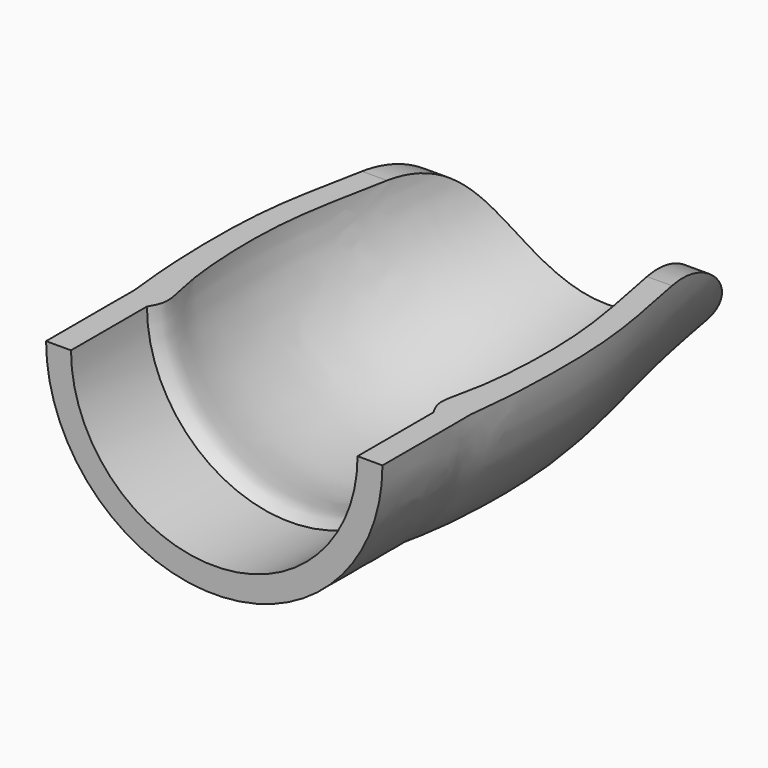
from build123d import *

# Parameters (mm, degrees)
F1_ANGLE    = 180
F2_T1_DEPTH = 235
F2_T3_DEPTH = 235


# Not quite as in the source:
# - a fillet or chamfer that OpenCascade refuses, or shapes differently, is made with other operations: its cross-section is extruded or revolved along the edge and cut away or added


with BuildPart() as f1:
    # F0 (on Top) → F1 (revolve)
    with BuildSketch(Plane.XY):
        with BuildLine():
            Line((55, 76.2), (45, 76.2))
            add(Edge.make_bspline(
                [(45, 76.2), (46.4314513107, 65.4743240031), (49.4342728448, 42.9745780396), (58.2913617327, 2.5444927944), (60.7679740967, -26.0894301808), (58.7809439185, -60.3358085831), (53.5427275811, -75.7766382868), (56.3670048957, -80.6107385976), (57.5, -82.55)],
                knots=[0, 0, 0, 0, 0.1935302552, 0.4059773556, 0.5886953586, 0.7831392141, 0.9130035116, 1, 1, 1, 1], degree=3))
            Line((57.5, -82.55), (57.5, -120.65))
            Line((57.5, -120.65), (67.5, -120.65))
            add(Edge.make_bspline(
                [(55, 76.2), (56.4448487865, 65.4735496208), (59.4077958305, 42.9708360316), (68.3641601176, 2.5594432328), (70.5377050341, -26.12710406), (69.5737841588, -60.0998956005), (67.2249671963, -76.0618392071), (67.611979836, -82.6108206706), (67.4592693335, -102.3954969726), (67.5036900604, -114.5662351269), (67.5, -120.65)],
                knots=[0, 0, 0, 0, 0.1503921233, 0.3154845037, 0.4574744391, 0.6084055945, 0.7088837212, 0.7740964569, 0.8870482285, 1, 1, 1, 1], degree=3))
        make_face()
    revolve(axis=Axis((0, 0, 0), (0, 1, 0)), revolution_arc=F1_ANGLE)

    # F2: fillet of radius 45 on 2 edges, made by hand

    # F2_s2 → F2_t1 (cut)
    with BuildSketch(Plane.YZ.offset(-67.5)):
        with BuildLine():
            ThreePointArc((76.2, -45), (63.0198051534, -13.1801948466), (31.2, 0))
            Line((31.2, 0), (76.2, 0))
            Line((76.2, 0), (76.2, -45))
        make_face()
    extrude(amount=F2_T1_DEPTH, mode=Mode.SUBTRACT)

    # F2_s4 → F2_t3 (cut)
    with BuildSketch(Plane.YZ.offset(-167.5)):
        with BuildLine():
            ThreePointArc((76.2, -45), (63.0198051534, -13.1801948466), (31.2, 0))
            Line((31.2, 0), (76.2, 0))
            Line((76.2, 0), (76.2, -45))
        make_face()
    extrude(amount=F2_T3_DEPTH, mode=Mode.SUBTRACT)


solid = f1.part
